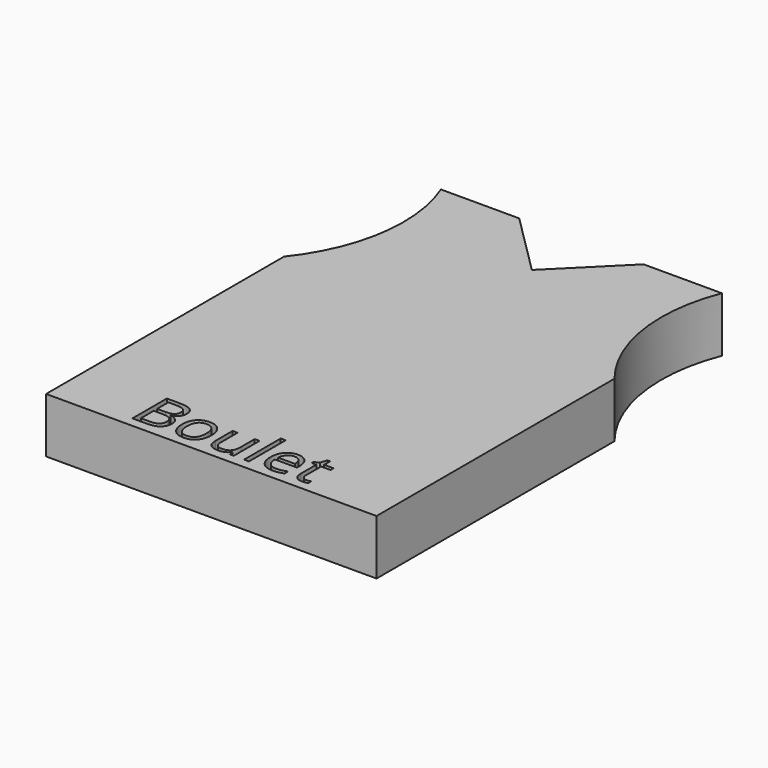
from build123d import *

# Parameters (mm, degrees)
F1_DEPTH     = 12.7
F2_TEXT_SIZE = 13.8915054914
F3_DEPTH     = 12.7
F4_TEXT_SIZE = 59.4727247894
F5_DEPTH     = 12.7


# Not quite as in the source:
# - Text() gives the source's letters only with a copy of the font that has no kerning and outlines rounded to 1/6400 em; it was checked with that copy


with BuildPart() as f1:
    # F0 (on Top) → F1 (new body)
    with BuildSketch(Plane.XY):
        with BuildLine():
            Line((-38.1, -3.048), (-38.1, -68.58))
            Line((-38.1, -68.58), (0, -68.58))
            Line((0, -68.58), (38.1, -68.58))
            Line((38.1, -68.58), (38.1, -3.048))
            ThreePointArc((38.1, -3.048), (27.5999430452, 16.223508368), (29.3496129293, 38.1))
            Line((29.3496129293, 38.1), (18.6458099633, 38.1))
            Line((18.6458099633, 38.1), (0, 19.5397089018))
            Line((0, 19.5397089018), (-18.6458099633, 38.1))
            Line((-18.6458099633, 38.1), (-29.3496129293, 38.1))
            ThreePointArc((-29.3496129293, 38.1), (-27.5999430452, 16.223508368), (-38.1, -3.048))
        make_face()
        with BuildLine():
            Line((-38.1, 0), (-38.1, -3.048))
            ThreePointArc((-38.1, -3.048), (-27.5999430452, 16.223508368), (-29.3496129293, 38.1))
            Line((-29.3496129293, 38.1), (-32.3976129293, 38.1))
            ThreePointArc((-32.3976129293, 38.1), (-30.1342936723, 18.2845162305), (-38.1, 0))
        make_face()
        with BuildLine():
            ThreePointArc((29.3496129293, 38.1), (27.5999430452, 16.223508368), (38.1, -3.048))
            Line((38.1, -3.048), (38.1, 0))
            ThreePointArc((38.1, 0), (30.1342936723, 18.2845162305), (32.3976129293, 38.1))
            Line((32.3976129293, 38.1), (29.3496129293, 38.1))
        make_face()
        Polygon((-14.3464950876, 38.1), (-18.6458099633, 38.1), (0, 19.5397089018), (18.6458099633, 38.1), (14.3464950876, 38.1), (0, 23.8193050027), align=None)
    extrude(amount=F1_DEPTH)

    # F2 (on Top) → F3 (cut)
    with BuildSketch(Plane.XY):
        with Locations((-21.3701277055, -66.3069480195)):
            Text('Boulet', F2_TEXT_SIZE, font='Open Sans', text_align=(TextAlign.LEFT, TextAlign.BOTTOM))
    extrude(amount=F3_DEPTH, mode=Mode.SUBTRACT)

    # F4 (on Top) → F5 (cut)
    with BuildSketch(Plane.XY):
        with Locations((-18.334325939, -44.4795419129)):
            Text('4', F4_TEXT_SIZE, font='Open Sans', text_align=(TextAlign.LEFT, TextAlign.BOTTOM))
    extrude(amount=-F5_DEPTH, mode=Mode.SUBTRACT)


solid = f1.part
